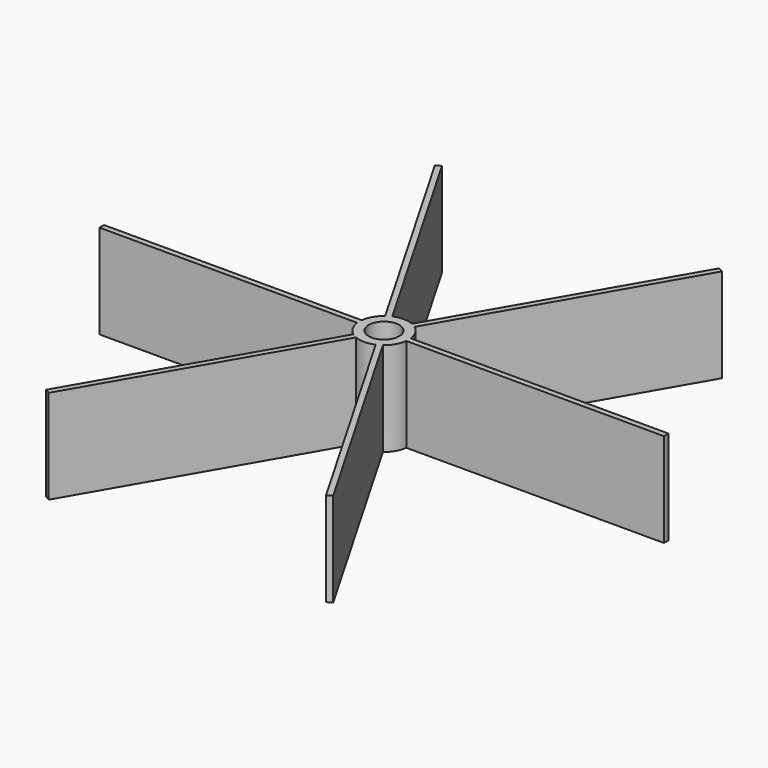
from build123d import *

# Parameters (mm, degrees)
F1_DEPTH = 20
F2_R     = 3.25
F3_DEPTH = 20.001


with BuildPart() as f1:
    # F0 (on Top) → F1 (new body)
    with BuildSketch(Plane.XY):
        with BuildLine():
            Line((-5.2141973622, 0.6), (-60, 0.6))
            Line((-60, 0.6), (-60, -0.6))
            Line((-60, -0.6), (-5.2141973622, -0.6))
            ThreePointArc((-5.2141973622, -0.6), (-5.2486049701, 0), (-5.2141973622, 0.6))
        make_face()
        with BuildLine():
            ThreePointArc((-3.1267139234, 4.215627376), (-4.5454252385, 2.624302485), (-5.2141973622, 0.6))
            Line((-5.2141973622, 0.6), (-1.0392304845, 0.6))
            Line((-1.0392304845, 0.6), (-3.1267139234, 4.215627376))
        make_face()
        with BuildLine():
            Line((-1.0392304845, 0.6), (-5.2141973622, 0.6))
            ThreePointArc((-5.2141973622, 0.6), (-5.2486049701, 0), (-5.2141973622, -0.6))
            Line((-5.2141973622, -0.6), (-1.0392304845, -0.6))
            Line((-1.0392304845, -0.6), (-0.692820323, 0))
            Line((-0.692820323, 0), (-1.0392304845, 0.6))
        make_face()
        with BuildLine():
            Line((-3.1267139234, 4.215627376), (-1.0392304845, 0.6))
            Line((-1.0392304845, 0.6), (-0.3464101615, 0.6))
            Line((-0.3464101615, 0.6), (0, 1.2))
            Line((0, 1.2), (-2.0874834388, 4.815627376))
            ThreePointArc((-2.0874834388, 4.815627376), (-2.624302485, 4.5454252385), (-3.1267139234, 4.215627376))
        make_face()
        with BuildLine():
            Line((-30.5196152423, 51.6615242271), (-3.1267139234, 4.215627376))
            ThreePointArc((-3.1267139234, 4.215627376), (-2.624302485, 4.5454252385), (-2.0874834388, 4.815627376))
            Line((-2.0874834388, 4.815627376), (-29.4803847577, 52.2615242271))
            Line((-29.4803847577, 52.2615242271), (-30.5196152423, 51.6615242271))
        make_face()
        with BuildLine():
            Line((-1.0392304845, -0.6), (-5.2141973622, -0.6))
            ThreePointArc((-5.2141973622, -0.6), (-4.5454252385, -2.624302485), (-3.1267139234, -4.215627376))
            Line((-3.1267139234, -4.215627376), (-1.0392304845, -0.6))
        make_face()
        with BuildLine():
            ThreePointArc((2.0874834388, 4.815627376), (0, 5.2486049701), (-2.0874834388, 4.815627376))
            Line((-2.0874834388, 4.815627376), (0, 1.2))
            Line((0, 1.2), (2.0874834388, 4.815627376))
        make_face()
        with BuildLine():
            Line((-0.3464101615, -0.6), (-1.0392304845, -0.6))
            Line((-1.0392304845, -0.6), (-3.1267139234, -4.215627376))
            ThreePointArc((-3.1267139234, -4.215627376), (-2.624302485, -4.5454252385), (-2.0874834388, -4.815627376))
            Line((-2.0874834388, -4.815627376), (0, -1.2))
            Line((0, -1.2), (-0.3464101615, -0.6))
        make_face()
        with BuildLine():
            ThreePointArc((-2.0874834388, -4.815627376), (-2.624302485, -4.5454252385), (-3.1267139234, -4.215627376))
            Line((-3.1267139234, -4.215627376), (-30.5196152423, -51.6615242271))
            Line((-30.5196152423, -51.6615242271), (-29.4803847577, -52.2615242271))
            Line((-29.4803847577, -52.2615242271), (-2.0874834388, -4.815627376))
        make_face()
        with BuildLine():
            Line((2.0874834388, 4.815627376), (0, 1.2))
            Line((0, 1.2), (0.3464101615, 0.6))
            Line((0.3464101615, 0.6), (1.0392304845, 0.6))
            Line((1.0392304845, 0.6), (3.1267139234, 4.215627376))
            ThreePointArc((3.1267139234, 4.215627376), (2.624302485, 4.5454252385), (2.0874834388, 4.815627376))
        make_face()
        with BuildLine():
            Line((29.4803847577, 52.2615242271), (2.0874834388, 4.815627376))
            ThreePointArc((2.0874834388, 4.815627376), (2.624302485, 4.5454252385), (3.1267139234, 4.215627376))
            Line((3.1267139234, 4.215627376), (30.5196152423, 51.6615242271))
            Line((30.5196152423, 51.6615242271), (29.4803847577, 52.2615242271))
        make_face()
        with BuildLine():
            Line((0, -1.2), (-2.0874834388, -4.815627376))
            ThreePointArc((-2.0874834388, -4.815627376), (0, -5.2486049701), (2.0874834388, -4.815627376))
            Line((2.0874834388, -4.815627376), (0, -1.2))
        make_face()
        with BuildLine():
            ThreePointArc((5.2141973622, 0.6), (4.5454252385, 2.624302485), (3.1267139234, 4.215627376))
            Line((3.1267139234, 4.215627376), (1.0392304845, 0.6))
            Line((1.0392304845, 0.6), (5.2141973622, 0.6))
        make_face()
        with BuildLine():
            Line((0.3464101615, -0.6), (0, -1.2))
            Line((0, -1.2), (2.0874834388, -4.815627376))
            ThreePointArc((2.0874834388, -4.815627376), (2.624302485, -4.5454252385), (3.1267139234, -4.215627376))
            Line((3.1267139234, -4.215627376), (1.0392304845, -0.6))
            Line((1.0392304845, -0.6), (0.3464101615, -0.6))
        make_face()
        with BuildLine():
            ThreePointArc((3.1267139234, -4.215627376), (2.624302485, -4.5454252385), (2.0874834388, -4.815627376))
            Line((2.0874834388, -4.815627376), (29.4803847577, -52.2615242271))
            Line((29.4803847577, -52.2615242271), (30.5196152423, -51.6615242271))
            Line((30.5196152423, -51.6615242271), (3.1267139234, -4.215627376))
        make_face()
        with BuildLine():
            Line((5.2141973622, 0.6), (1.0392304845, 0.6))
            Line((1.0392304845, 0.6), (0.692820323, 0))
            Line((0.692820323, 0), (1.0392304845, -0.6))
            Line((1.0392304845, -0.6), (5.2141973622, -0.6))
            ThreePointArc((5.2141973622, -0.6), (5.2399960077, -0.3004928799), (5.2486049701, 0))
            ThreePointArc((5.2486049701, 0), (5.2399960077, 0.3004928799), (5.2141973622, 0.6))
        make_face()
        with BuildLine():
            Line((60, 0.6), (5.2141973622, 0.6))
            ThreePointArc((5.2141973622, 0.6), (5.2399960077, 0.3004928799), (5.2486049701, 0))
            ThreePointArc((5.2486049701, 0), (5.2399960077, -0.3004928799), (5.2141973622, -0.6))
            Line((5.2141973622, -0.6), (60, -0.6))
            Line((60, -0.6), (60, 0.6))
        make_face()
        with BuildLine():
            Line((1.0392304845, -0.6), (3.1267139234, -4.215627376))
            ThreePointArc((3.1267139234, -4.215627376), (4.5454252385, -2.624302485), (5.2141973622, -0.6))
            Line((5.2141973622, -0.6), (1.0392304845, -0.6))
        make_face()
    extrude(amount=F1_DEPTH)

    # F2 (on face) → F3 (cut, through all)
    with BuildSketch(Plane.XY.offset(20)):
        Circle(F2_R)
        Polygon((1.0392304845, 0.6), (0.692820323, 0), (1.0392304845, -0.6), (0.3464101615, -0.6), (0, -1.2), (-0.3464101615, -0.6), (-1.0392304845, -0.6), (-0.692820323, 0), (-1.0392304845, 0.6), (-0.3464101615, 0.6), (0, 1.2), (0.3464101615, 0.6), align=None, mode=Mode.SUBTRACT)
    extrude(amount=-F3_DEPTH, mode=Mode.SUBTRACT)


solid = f1.part
